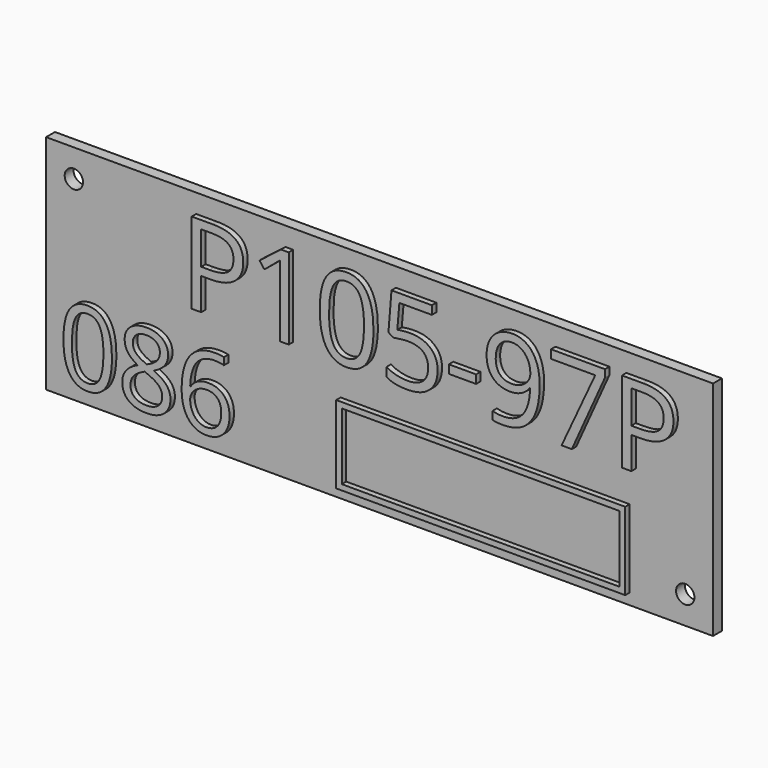
from build123d import *

# Parameters (mm, degrees)
F0_W         = 120
F0_H         = 40
F1_DEPTH     = 2
F3_D         = 3.3
F4_TEXT_SIZE = 20.4639926102
F5_DEPTH     = 1
F6_TEXT_SIZE = 18.4837545126
F7_DEPTH     = 1
F8_W         = 52
F8_H         = 14
F8_W_2       = 49.99999962
F8_H_2       = 11.99999962
F9_DEPTH     = 1


# Not quite as in the source:
# - Text() gives the source's letters only with a copy of the font that has no kerning and outlines rounded to 1/6400 em; it was checked with that copy


with BuildPart() as f1:
    # F0 (on Front) → F1 (new body)
    with BuildSketch(Plane.XZ):
        Rectangle(F0_W, F0_H)
    extrude(amount=F1_DEPTH)

    # F3 (through all)
    with Locations(Plane.XZ.offset(2)):
        with Locations((-55, 15), (55, -15)):
            Hole(F3_D / 2)

    # F4 (on face) → F5 (join)
    with BuildSketch(Plane.XZ.offset(2)):
        with Locations((-35, 2)):
            Text('P105-97P', F4_TEXT_SIZE, font='Open Sans', text_align=(TextAlign.LEFT, TextAlign.BOTTOM))
    extrude(amount=F5_DEPTH)

    # F6 (on face) → F7 (join)
    with BuildSketch(Plane.XZ.offset(2)):
        with Locations((-57, -17)):
            Text('086', F6_TEXT_SIZE, font='Open Sans', text_align=(TextAlign.LEFT, TextAlign.BOTTOM))
    extrude(amount=F7_DEPTH)

    # F8 (on face) → F9 (join)
    with BuildSketch(Plane.XZ.offset(2)):
        with Locations((19, -11)):
            Rectangle(F8_W, F8_H)
        with Locations((19, -11)):
            Rectangle(F8_W_2, F8_H_2, mode=Mode.SUBTRACT)
    extrude(amount=F9_DEPTH)


solid = f1.part
